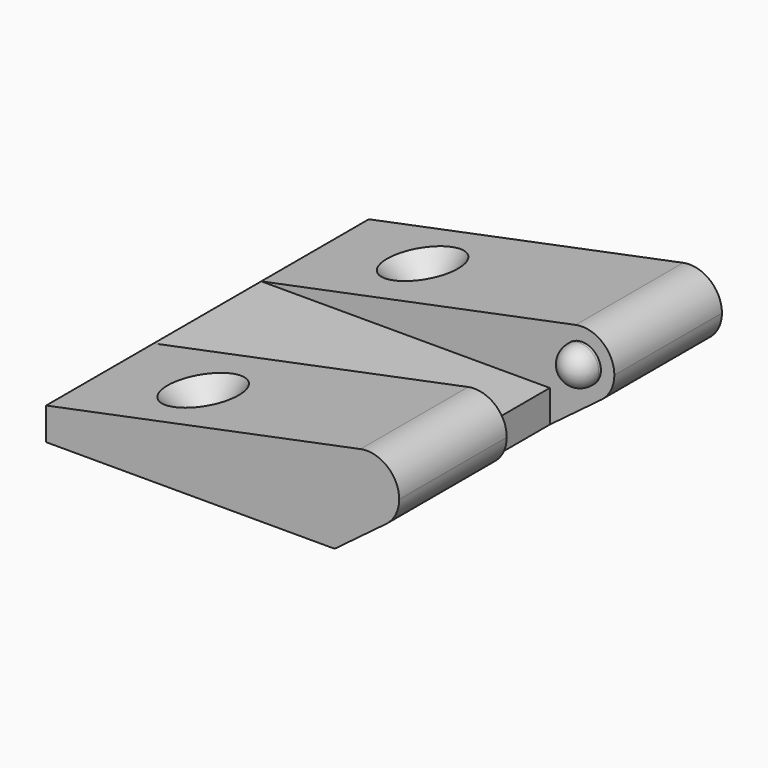
from build123d import *

# Parameters (mm, degrees)
F0_W            = 53.6510385573
F0_H            = 6
F0_R            = 3
F1_DEPTH        = 37.5
F1_DEPTH_BACK   = 37.5
F3_DEPTH        = 12.5
F3_DEPTH_BACK   = 12.5
F4_R            = 3.5
F5_DEPTH        = 4
F6_R            = 3.5
F7_DEPTH        = 4
F8_R            = 3.5
F10_D           = 6.7564
F10_CSINK_D     = 13.4874
F10_CSINK_ANGLE = 82


# Not quite as in the source:
# - a feature of the source that left no trace in its solid (it failed there, or was rolled back) is left out


with BuildPart() as f1:
    # F0 (on Front) → F1 (new body, two sides)
    with BuildSketch(Plane.XZ) as f1_sk:
        with Locations((-26.8255192786, 3)):
            Rectangle(F0_W, F0_H)
        with BuildLine():
            Line((0, 6), (0, 0))
            Line((0, 0), (9.6, 7.2))
            ThreePointArc((9.6, 7.2), (0.5263664708, 9.5424939495), (4.8050694646, 17.8798079064))
            Line((4.8050694646, 17.8798079064), (-53.6510385573, 6))
            Line((-53.6510385573, 6), (0, 6))
        make_face()
        with BuildLine():
            ThreePointArc((4.8050694646, 17.8798079064), (0.5263664708, 9.5424939495), (9.6, 7.2))
            ThreePointArc((9.6, 7.2), (11.366563146, 9.316718427), (12, 12))
            ThreePointArc((12, 12), (9.7967365452, 16.6459435647), (4.8050694646, 17.8798079064))
        make_face()
        with Locations((6, 12)):
            Circle(F0_R, mode=Mode.SUBTRACT)
        with Locations((6, 12)):
            Circle(F0_R)
    extrude(amount=F1_DEPTH)
    extrude(f1_sk.sketch, amount=-F1_DEPTH_BACK)

    # F0 (on Front) → F3 (cut, two sides)
    with BuildSketch(Plane.XZ) as f3_sk:
        with BuildLine():
            Line((0, 6), (0, 0))
            Line((0, 0), (9.6, 7.2))
            ThreePointArc((9.6, 7.2), (0.5263664708, 9.5424939495), (4.8050694646, 17.8798079064))
            Line((4.8050694646, 17.8798079064), (-53.6510385573, 6))
            Line((-53.6510385573, 6), (0, 6))
        make_face()
        with BuildLine():
            ThreePointArc((4.8050694646, 17.8798079064), (0.5263664708, 9.5424939495), (9.6, 7.2))
            ThreePointArc((9.6, 7.2), (11.366563146, 9.316718427), (12, 12))
            ThreePointArc((12, 12), (9.7967365452, 16.6459435647), (4.8050694646, 17.8798079064))
        make_face()
        with Locations((6, 12)):
            Circle(F0_R, mode=Mode.SUBTRACT)
        with Locations((6, 12)):
            Circle(F0_R)
    extrude(amount=F3_DEPTH, mode=Mode.SUBTRACT)
    extrude(f3_sk.sketch, amount=-F3_DEPTH_BACK, mode=Mode.SUBTRACT)

    # F4 (on face) → F5 (join)
    with BuildSketch(Plane.XZ.offset(-12.5)):
        with Locations((6, 12)):
            Circle(F4_R)
    extrude(amount=F5_DEPTH)

    # F6 (on face) → F7 (join)
    with BuildSketch(Plane(origin=(0, -12.5, 0), x_dir=(-1, 0, 0), z_dir=(0, 1, 0))):
        with Locations((-6, 12)):
            Circle(F6_R)
    extrude(amount=F7_DEPTH)

    # F8
    f8_edges = [f1.edges().sort_by_distance(p)[0] for p in [
        (9.5, -8.5, 12),
        (2.5, 8.5, 12),
    ]]
    fillet(f8_edges, radius=F8_R)

    # F10 (through all)
    with Locations(Plane(origin=(-3.2989413744, 0, 16.2328612433), x_dir=(0.9799679844, 0, 0.1991550892), z_dir=(-0.1991550892, 0, 0.9799679844))):
        with Locations((-31.3813695802, -25.5), (-31.3813695802, 25.5)):
            CounterSinkHole(F10_D / 2, F10_CSINK_D / 2, counter_sink_angle=F10_CSINK_ANGLE)


solid = f1.part
